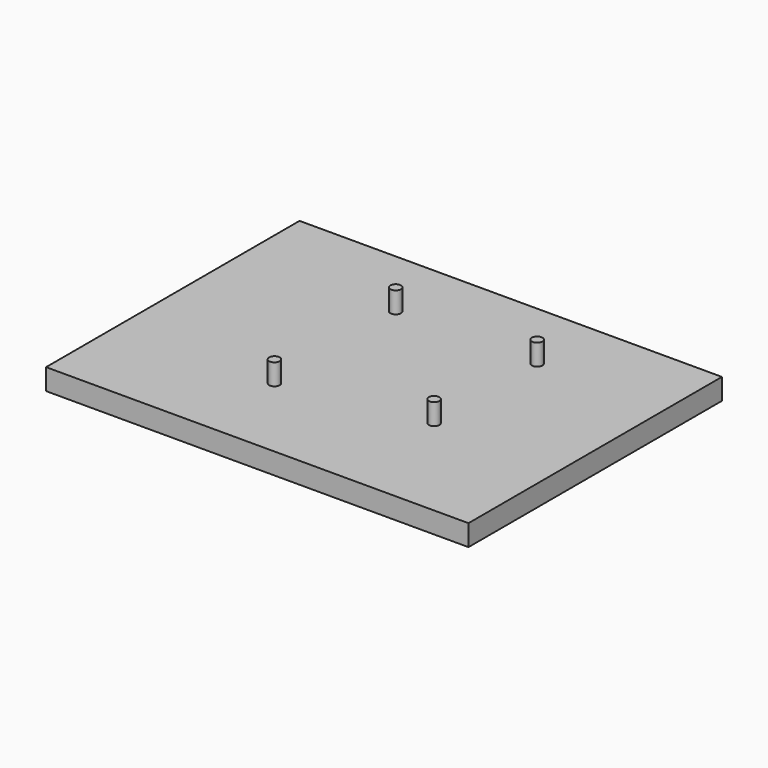
from build123d import *

# Parameters (mm, degrees)
F0_W       = 508
F0_H       = 381
F1_DEPTH   = 25.4
F2_R       = 6.35
F3_DEPTH   = 25.4
F1_FACE1_W = 508
F1_FACE1_H = 381
F4_DEPTH   = 25.4
F5_DEPTH   = 25.4


# Not quite as in the source:
# - a feature names something its author has since deleted; it is built from what else it names


with BuildPart() as f1:
    # F0 (on Top) → F1 (new body)
    with BuildSketch(Plane.XY):
        with Locations((15.942402184, 51.6951617887)):
            Rectangle(F0_W, F0_H)
    extrude(amount=F1_DEPTH)

    # F2 (on face) → F3 (join)
    with BuildSketch(Plane.XY.offset(25.4)):
        with Locations((-52.637597816, 154.94)):
            Circle(F2_R)
        with Locations((117.542402184, 154.94)):
            Circle(F2_R)
        with Locations((117.542402184, 0)):
            Circle(F2_R)
    extrude(amount=F3_DEPTH)

    # F2 (on face) + F1_face1 (on face) → F4 (join)
    with BuildSketch(Plane.XY.offset(25.4)):
        with Locations((-52.637597816, 154.94)):
            Circle(F2_R)
        with Locations((117.542402184, 154.94)):
            Circle(F2_R)
        with Locations((117.542402184, 0)):
            Circle(F2_R)
        with Locations((-50.097597816, -30.48)):
            Circle(F2_R)
    with BuildSketch(Plane(origin=(15.942402184, 51.6951617887, 0), x_dir=(1, 0, 0), z_dir=(0, 0, -1))):
        Rectangle(F1_FACE1_W, F1_FACE1_H)
    extrude(amount=F4_DEPTH, dir=(0, 0, 1))

    # F2 (on face) + F1_face1 (on face) → F5 (join)
    with BuildSketch(Plane.XY.offset(25.4)):
        with Locations((-52.637597816, 154.94)):
            Circle(F2_R)
        with Locations((117.542402184, 154.94)):
            Circle(F2_R)
        with Locations((117.542402184, 0)):
            Circle(F2_R)
        with Locations((-50.097597816, -30.48)):
            Circle(F2_R)
    with BuildSketch(Plane(origin=(15.942402184, 51.6951617887, 0), x_dir=(1, 0, 0), z_dir=(0, 0, -1))):
        Rectangle(F1_FACE1_W, F1_FACE1_H)
    extrude(amount=F5_DEPTH, dir=(0, 0, 1))


solid = f1.part
